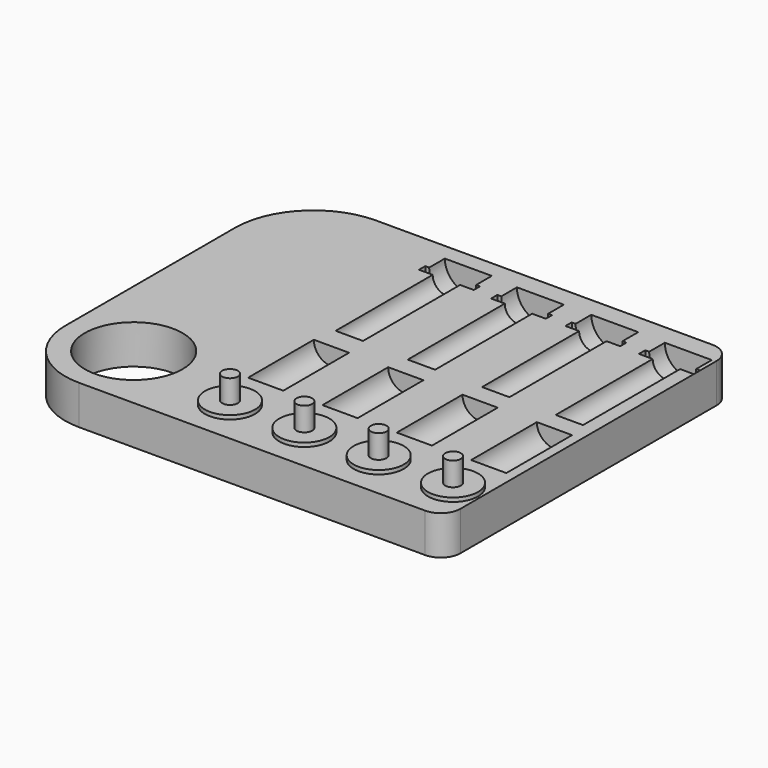
from build123d import *

# Parameters (mm, degrees)
F0_R         = 12.5
F1_DEPTH     = 10
F2_W         = 4.5
F2_H         = 21
F2_R         = 6.4
F2_R_2       = 2
F7_DEPTH     = 1
F8_DEPTH     = 7
F9_TEXT_SIZE = 6.9444444444
F10_DEPTH    = 1


# Not quite as in the source:
# - Text() gives the source's letters only with a copy of the font that has no kerning and outlines rounded to 1/6400 em; it was checked with that copy


with BuildPart() as f1:
    # F0 (on Top) → F1 (new body)
    with BuildSketch(Plane.XY):
        with BuildLine():
            ThreePointArc((0, 17.5), (5.1256313292, 5.1256313292), (17.5, 0))
            Line((17.5, 0), (106, 0))
            ThreePointArc((106, 0), (109.5355339059, 1.4644660941), (111, 5))
            Line((111, 5), (111, 86.8))
            ThreePointArc((111, 86.8), (109.5355339059, 90.3355339059), (106, 91.8))
            Line((106, 91.8), (20, 91.8))
            ThreePointArc((20, 91.8), (5.8578643763, 85.9421356237), (0, 71.8))
            Line((0, 71.8), (0, 17.5))
        make_face()
        with Locations((17.5, 17.5)):
            Circle(F0_R, mode=Mode.SUBTRACT)
    extrude(amount=F1_DEPTH)

    # F2 (on face) → F3 (revolve, cut)
    with BuildSketch(Plane.XY.offset(10)):
        Polygon((47, 80.5231896639), (47, 49.5231896639), (50.5, 49.5231896639), (50.5, 80.5231896639), (54, 80.5231896639), (54, 82.5231896639), (53, 82.5231896639), (53, 87.5231896639), (47, 87.5231896639), (47, 82.5231896639), align=None)
        with Locations((49.25, 33.3)):
            Rectangle(F2_W, F2_H)
    revolve(axis=Axis((47, 33.3, 10), (0, 1, 0)), mode=Mode.SUBTRACT)

    # F2 (on face) → F4 (revolve, cut)
    with BuildSketch(Plane.XY.offset(10)):
        Polygon((66, 79.8), (66, 48.8), (69.5, 48.8), (69.5, 79.8), (73, 79.8), (73, 81.8), (72, 81.8), (72, 86.8), (66, 86.8), (66, 81.8), align=None)
        with Locations((68.25, 33.3)):
            Rectangle(F2_W, F2_H)
    revolve(axis=Axis((66, 33.3, 10), (0, 1, 0)), mode=Mode.SUBTRACT)

    # F2 (on face) → F5 (revolve, cut)
    with BuildSketch(Plane.XY.offset(10)):
        Polygon((85, 79.8), (85, 48.8), (88.5, 48.8), (88.5, 79.8), (92, 79.8), (92, 81.8), (91, 81.8), (91, 86.8), (85, 86.8), (85, 81.8), align=None)
        with Locations((87.25, 33.3)):
            Rectangle(F2_W, F2_H)
    revolve(axis=Axis((85, 33.3, 10), (0, 1, 0)), mode=Mode.SUBTRACT)

    # F2 (on face) → F6 (revolve, cut)
    with BuildSketch(Plane.XY.offset(10)):
        Polygon((104, 79.552416265), (104, 48.552416265), (107.5, 48.552416265), (107.5, 79.552416265), (111, 79.552416265), (111, 81.552416265), (110, 81.552416265), (110, 86.552416265), (104, 86.552416265), (104, 81.552416265), align=None)
        with Locations((106.25, 33.3)):
            Rectangle(F2_W, F2_H)
    revolve(axis=Axis((104, 64.052416265, 10), (0, 1, 0)), mode=Mode.SUBTRACT)

    # F2 (on face) → F7 (join)
    with BuildSketch(Plane.XY.offset(10)):
        with Locations((47, 11.4)):
            Circle(F2_R)
        with Locations((47, 11.4)):
            Circle(F2_R_2, mode=Mode.SUBTRACT)
        with Locations((66, 11.4)):
            Circle(F2_R)
        with Locations((66, 11.4)):
            Circle(F2_R_2, mode=Mode.SUBTRACT)
        with Locations((85, 11.4)):
            Circle(F2_R)
        with Locations((85, 11.4)):
            Circle(F2_R_2, mode=Mode.SUBTRACT)
        with Locations((104, 11.4)):
            Circle(F2_R)
        with Locations((104, 11.4)):
            Circle(F2_R_2, mode=Mode.SUBTRACT)
    extrude(amount=F7_DEPTH)

    # F2 (on face) → F8 (join)
    with BuildSketch(Plane.XY.offset(10)):
        with Locations((66, 11.4)):
            Circle(F2_R_2)
        with Locations((47, 11.4)):
            Circle(F2_R_2)
        with Locations((85, 11.4)):
            Circle(F2_R_2)
        with Locations((104, 11.4)):
            Circle(F2_R_2)
    extrude(amount=F8_DEPTH)

    # F9 (on face) → F10 (cut)
    with BuildSketch(Plane(origin=(0, 0, 0), x_dir=(1, 0, 0), z_dir=(0, 0, -1))):
        with Locations((30, -10)):
            Text('1060', F9_TEXT_SIZE, font='Open Sans', text_align=(TextAlign.LEFT, TextAlign.BOTTOM))
    extrude(amount=-F10_DEPTH, mode=Mode.SUBTRACT)


solid = f1.part
